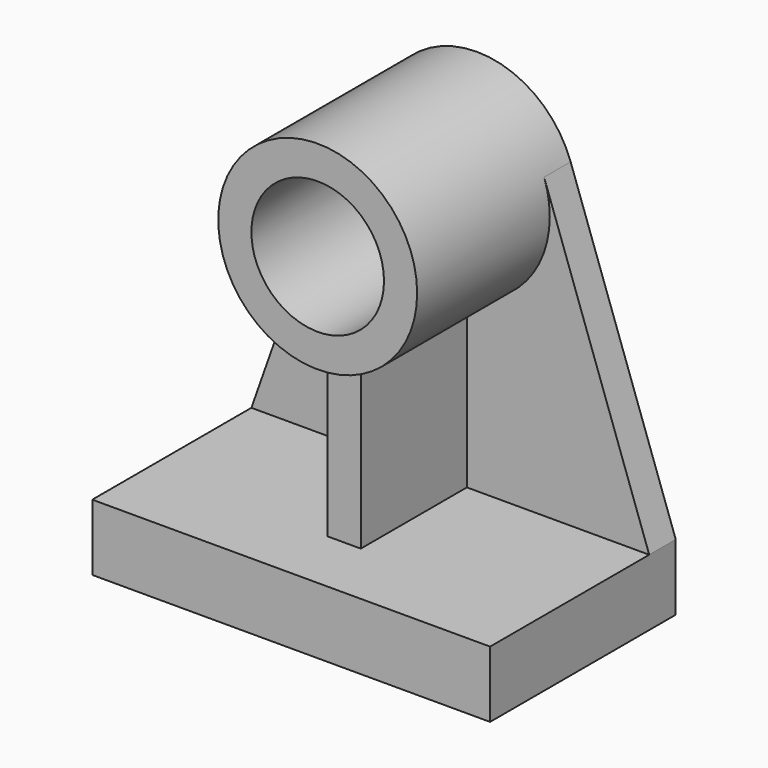
from build123d import *

# Parameters (mm, degrees)
F2_DEPTH  = 25.4
F3_W      = 304.8
F3_H      = 50.8
F4_DEPTH  = 152.4
F5_W      = 25.4
F5_H      = 203.2
F6_DEPTH  = 101.6
F7_R      = 76.2
F8_DEPTH  = 127
F9_R      = 50.8
F10_DEPTH = 152.401


# Not quite as in the source:
# - a variable given as a bare number and used for a length is read in inches; the dataset says mm whatever the document's units were


with BuildPart() as f2:
    # F1 (on Front) → F2 (new body)
    with BuildSketch(Plane.XZ):
        with BuildLine():
            Line((-304.8, 0), (0, 0))
            Line((0, 0), (0, 50.8))
            Line((0, 50.8), (-80.5318662816, 279.3261002888))
            ThreePointArc((-80.5318662816, 279.3261002888), (-152.4, 330.2), (-224.2681337184, 279.3261002888))
            Line((-224.2681337184, 279.3261002888), (-304.8, 50.8))
            Line((-304.8, 50.8), (-304.8, 0))
        make_face()
    extrude(amount=F2_DEPTH)

    # F3 (on face) → F4 (join)
    with BuildSketch(Plane.XZ.offset(25.4)):
        with Locations((-152.4, 25.4)):
            Rectangle(F3_W, F3_H)
    extrude(amount=F4_DEPTH)

    # F5 (on face) → F6 (join)
    with BuildSketch(Plane.XZ.offset(25.4)):
        with Locations((-152.4, 152.4)):
            Rectangle(F5_W, F5_H)
    extrude(amount=F6_DEPTH)

    # F7 (on face) → F8 (join)
    with BuildSketch(Plane.XZ.offset(25.4)):
        with Locations((-152.4, 254)):
            Circle(F7_R)
    extrude(amount=F8_DEPTH)

    # F9 (on face) → F10 (cut, through all)
    with BuildSketch(Plane.XZ.offset(152.4)):
        with Locations((-152.4, 254)):
            Circle(F9_R)
    extrude(amount=-F10_DEPTH, mode=Mode.SUBTRACT)


solid = f2.part
